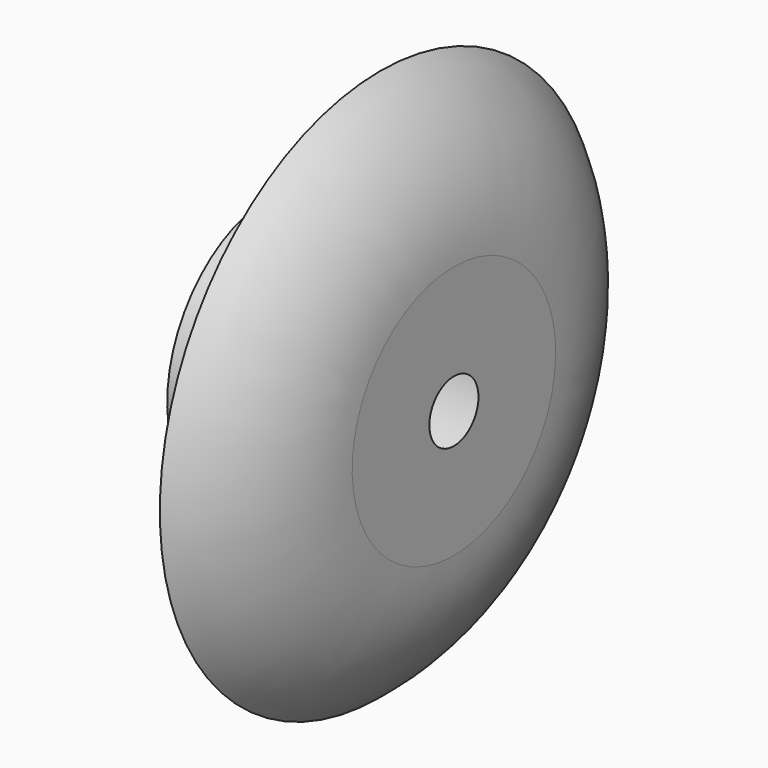
from build123d import *

# Parameters (mm, degrees)
F4_D     = 5
F4_DEPTH = 4
F4_TIP   = 1.5021515476


# Not quite as in the source:
# - a fillet or chamfer that OpenCascade refuses, or shapes differently, is made with other operations: its cross-section is extruded or revolved along the edge and cut away or added


with BuildPart() as f3:
    # F0 (on Front) → F3 (revolve)
    with BuildSketch(Plane.XZ):
        Polygon((3, 3.5), (0, 3.5), (0, 0), (5, 0), (5, 7.5), (3, 7.5), align=None)
    revolve(axis=Axis((2.5, 0, 0), (-1, 0, 0)))

    # F4
    with Locations(Plane(origin=(0, 0, 0), x_dir=(0, -1, 0), z_dir=(-1, 0, 0))):
        with Locations((0, 0)):
            Hole(F4_D / 2, depth=F4_DEPTH)
            with Locations((0, 0, -(F4_DEPTH + F4_TIP / 2))):  # 118° drill point
                Cone(0, F4_D / 2, F4_TIP, mode=Mode.SUBTRACT)

    # F2: fillet of radius 5.08 on 1 edges, made by hand

    # F2_s1 → F2_t2 (revolve, cut)
    with BuildSketch(Plane.XZ):
        with BuildLine():
            ThreePointArc((3, 7.5), (4.4726256161, 5.7140835586), (5, 3.4601980247))
            Line((5, 3.4601980247), (5, 7.5))
            Line((5, 7.5), (3, 7.5))
        make_face()
    revolve(axis=Axis((5, 0, 0), (-1, 0, 0)), mode=Mode.SUBTRACT)


solid = f3.part
